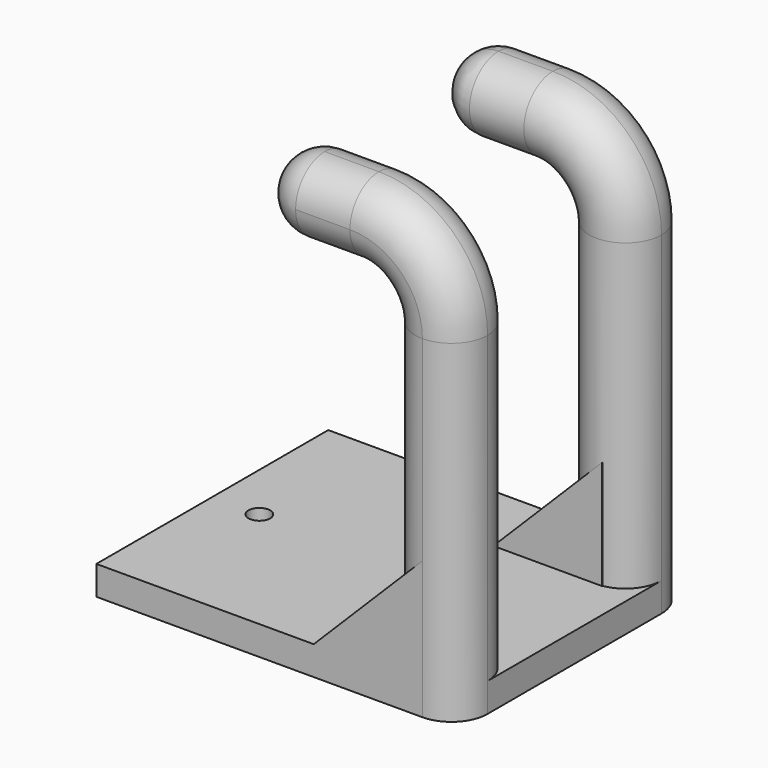
from build123d import *
from build123d import SkipClean  # not in build123d's __all__

# Parameters (mm, degrees)
F0_W      = 50
F0_H      = 40
F0_R      = 1.5
F1_DEPTH  = 4
F2_R      = 3.25
F9_R      = 5
F10_DEPTH = 2.5
F12_R     = 5
F13_DEPTH = 2.5
F14_R     = 4.9999
F17_DEPTH = 10
F18_DEPTH = 25
F20_DEPTH = 10


# Not quite as in the source:
# - a fillet or chamfer that OpenCascade refuses, or shapes differently, is made with other operations: its cross-section is extruded or revolved along the edge and cut away or added
# - a fillet or chamfer is up to 0.001 mm smaller than in the source, because OpenCascade refuses the exact size


with BuildPart() as f1:
    # F0 (on Top) → F1 (new body)
    with BuildSketch(Plane.XY):
        Rectangle(F0_W, F0_H)
        with Locations((-18.505550921, 0)):
            Circle(F0_R, mode=Mode.SUBTRACT)
    extrude(amount=F1_DEPTH)

    # F5: sweep along a path in F4
    with BuildLine(Plane.XZ.offset(-15)) as f5_path:
        Line((20, 4), (20, 46))
        ThreePointArc((20, 46), (17.0710678119, 53.0710678119), (10, 56))
        Line((10, 56), (0, 56))
    # F2 (on face) → F5 (sweep)
    with BuildSketch(Plane.XY.offset(4)):
        with BuildLine():
            ThreePointArc((20, 20), (16.4644660941, 11.4644660941), (25, 15))
            ThreePointArc((25, 15), (23.5355339059, 18.5355339059), (20, 20))
        make_face()
        with Locations((20, 15)):
            Circle(F2_R, mode=Mode.SUBTRACT)
    sweep(path=f5_path.line)

    # F8: sweep along a path in F7
    with BuildLine(Plane.XZ.offset(15)) as f8_path:
        Line((20, 4), (20, 46))
        ThreePointArc((20, 46), (17.0710678119, 53.0710678119), (10, 56))
        Line((10, 56), (0, 56))
    # F2 (on face) → F8 (sweep)
    with BuildSketch(Plane.XY.offset(4)):
        with BuildLine():
            ThreePointArc((19.9999999389, -20), (23.5355338843, -18.5355339275), (25, -15))
            ThreePointArc((25, -15), (16.4644661157, -11.4644660725), (19.9999999389, -20))
        make_face()
        with Locations((20, -15)):
            Circle(F2_R, mode=Mode.SUBTRACT)
    sweep(path=f8_path.line)

    # F9 (on face) → F10 (join)
    with BuildSketch(Plane(origin=(0, 0, 0), x_dir=(0, -1, 0), z_dir=(-1, 0, 0))):
        with Locations((15, 56)):
            Circle(F9_R)
    extrude(amount=F10_DEPTH)

    # F11: fillet of radius 5 on 1 edges, made by hand

    # F11_s1 → F11_t2 (revolve, cut)
    with BuildSketch(Plane.XY.offset(56)):
        with BuildLine():
            ThreePointArc((2.5, -20), (-1.0355339059, -18.5355339059), (-2.5, -15))
            Line((-2.5, -15), (-2.5, -20))
            Line((-2.5, -20), (2.5, -20))
        make_face()
    revolve(axis=Axis((-2.5, -15, 56), (-1, 0, 0)), mode=Mode.SUBTRACT)

    # F12 (on face) → F13 (join)
    with BuildSketch(Plane(origin=(0, 0, 0), x_dir=(0, -1, 0), z_dir=(-1, 0, 0))):
        with Locations((-15, 56)):
            Circle(F12_R)
    extrude(amount=F13_DEPTH)

    # F14 (radius 5 in the source; OpenCascade refuses exactly that, so slightly less here)
    f14_edges = [f1.edges().sort_by_distance(p)[0] for p in [
        (-2.5, 20, 56),
        (25, 20, 2),
        (25, -20, 2),
    ]]
    fillet(f14_edges, radius=F14_R)

    # F16 (on offset) → F17 (join)
    with BuildSketch(Plane(origin=(0, 10, 0), x_dir=(-1, 0, 0), z_dir=(0, 1, 0))):
        Polygon((-20.7827799022, 4), (-5.7827799022, 4), (-20.7827799022, 19), align=None)
    with SkipClean():  # cleaning this boolean's faces spoils the solid; the shape is the same uncleaned
        extrude(amount=F17_DEPTH)

    # F2 (on face) → F18 (cut)
    with BuildSketch(Plane.XY.offset(4)):
        with BuildLine():
            Line((25, -20), (25, -15))
            ThreePointArc((25, -15), (23.5355338843, -18.5355339275), (19.9999999389, -20))
            Line((19.9999999389, -20), (25, -20))
        make_face()
        with BuildLine():
            ThreePointArc((20, 20), (23.5355339059, 18.5355339059), (25, 15))
            Line((25, 15), (25, 20))
            Line((25, 20), (20, 20))
        make_face()
    extrude(amount=-F18_DEPTH, mode=Mode.SUBTRACT)

    # F19 (on face) → F20 (join)
    with BuildSketch(Plane.XZ.offset(20)):
        Polygon((5, 4), (20, 4), (20, 19), align=None)
    extrude(amount=-F20_DEPTH)


solid = f1.part
